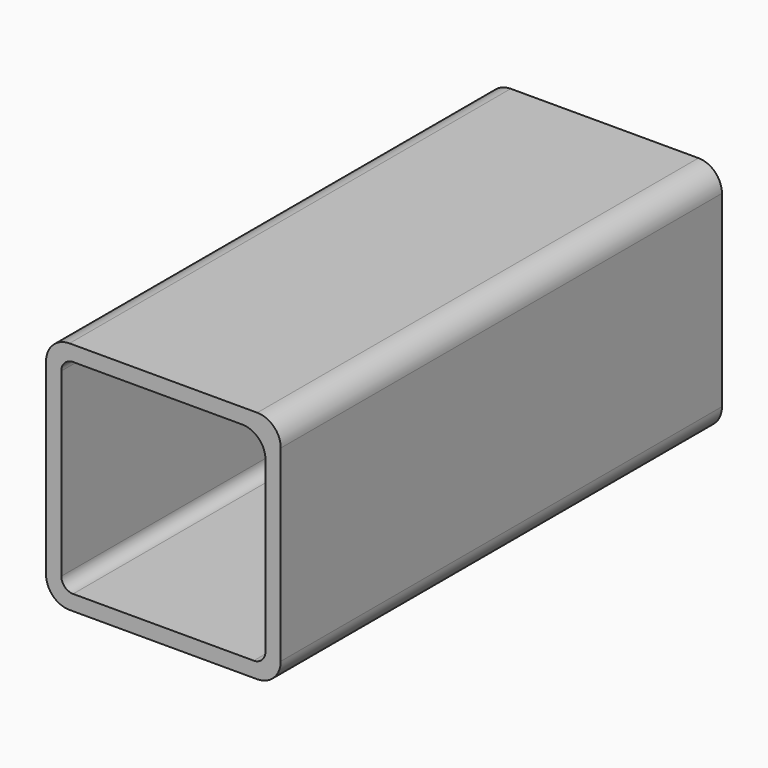
from build123d import *

# Parameters (mm, degrees)
F0_W     = 40
F0_H     = 40
F0_W_2   = 34.8
F0_H_2   = 34.8
F1_DEPTH = 94
F2_R     = 4
F3_R     = 2


with BuildPart() as f1:
    # F0 (on Front) → F1 (new body)
    with BuildSketch(Plane.XZ):
        Rectangle(F0_W, F0_H)
        Rectangle(F0_W_2, F0_H_2, mode=Mode.SUBTRACT)
    extrude(amount=F1_DEPTH)

    # F2
    f2_edges = [f1.edges().sort_by_distance(p)[0] for p in [
        (20, -47, 20),
        (-20, -47, 20),
        (20, -47, -20),
        (-20, -47, -20),
        (17.4, -47, 17.4),
    ]]
    fillet(f2_edges, radius=F2_R)

    # F3
    f3_edges = [f1.edges().sort_by_distance(p)[0] for p in [
        (-17.4, -47, 17.4),
        (-17.4, -47, -17.4),
        (17.4, -47, -17.4),
        (16, -47, 20),
    ]]
    fillet(f3_edges, radius=F3_R)


solid = f1.part
